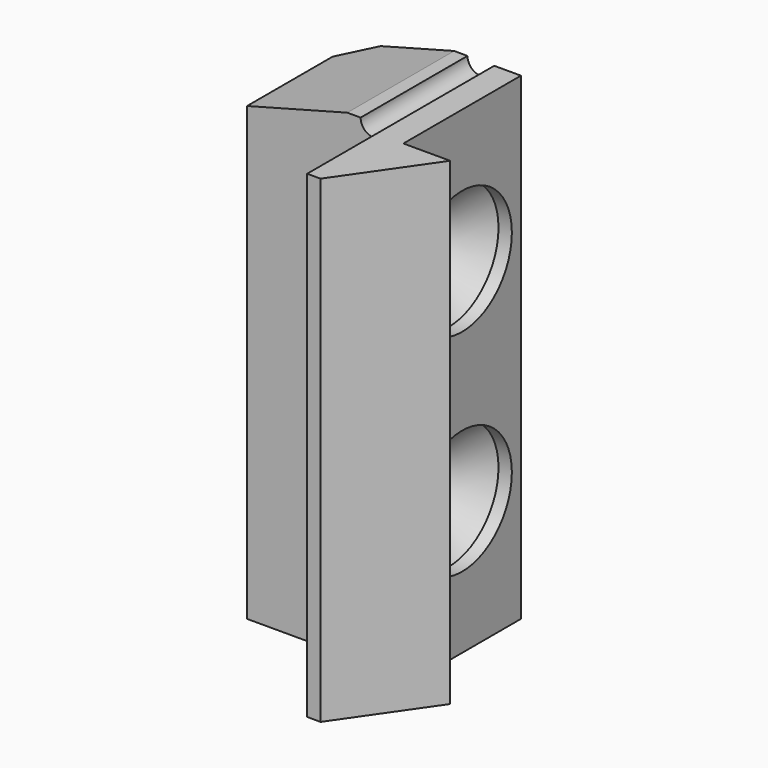
from build123d import *

# Parameters (mm, degrees)
F1_DEPTH = 40
F3_DEPTH = 12.5
F4_R     = 2.2
F5_DEPTH = 12.501
F7_SIZE  = 2
F6_R     = 4.65
F8_DEPTH = 1
F9_SIZE  = 2.44999


# Not quite as in the source:
# - a fillet or chamfer is up to 0.001 mm smaller than in the source, because OpenCascade refuses the exact size


with BuildPart() as f1:
    # F0 (on Top) → F1 (new body)
    with BuildSketch(Plane.XY):
        Polygon((2, 10), (-10.5, 10), (-10.5, 0), (0, 0), (0, -7.5), (1, -7.5), (5.5, -1), (2, -1), align=None)
    extrude(amount=F1_DEPTH)

    # F2 (on face) → F3 (cut, symmetric)
    with BuildSketch(Plane.XZ):
        with BuildLine():
            ThreePointArc((-2, 35.8), (-1, 34.8), (0, 35.8))
            Line((0, 35.8), (5.5, 35.8))
            Line((5.5, 35.8), (5.5, 40))
            Line((5.5, 40), (-10.5, 40))
            Line((-10.5, 40), (-10.5, 33.8))
            Line((-10.5, 33.8), (-3, 35.8))
            Line((-3, 35.8), (-2, 35.8))
        make_face()
    extrude(amount=F3_DEPTH, both=True, mode=Mode.SUBTRACT)

    # F4 (on face) → F5 (cut, through all)
    with BuildSketch(Plane.YZ.offset(2)):
        with Locations((4.5, 25.8)):
            Circle(F4_R)
        with Locations((4.5, 10)):
            Circle(F4_R)
    extrude(amount=-F5_DEPTH, mode=Mode.SUBTRACT)

    # F7
    f7_edges = [f1.edges().sort_by_distance(p)[0] for p in [
        (-10.5, 10, 16.9),
    ]]
    chamfer(f7_edges, length=F7_SIZE)

    # F6 (on face) → F8 (cut)
    with BuildSketch(Plane.YZ.offset(2)):
        with Locations((4.5, 25.8)):
            Circle(F6_R)
        with Locations((4.5, 10)):
            Circle(F6_R)
    extrude(amount=-F8_DEPTH, mode=Mode.SUBTRACT)

    # F9 (size 2.45 in the source; OpenCascade refuses exactly that, so slightly less here)
    f9_edges = [f1.edges().sort_by_distance(p)[0] for p in [
        (1, 2.3, 25.8),
        (1, 2.3, 10),
    ]]
    chamfer(f9_edges, length=F9_SIZE)


solid = f1.part
